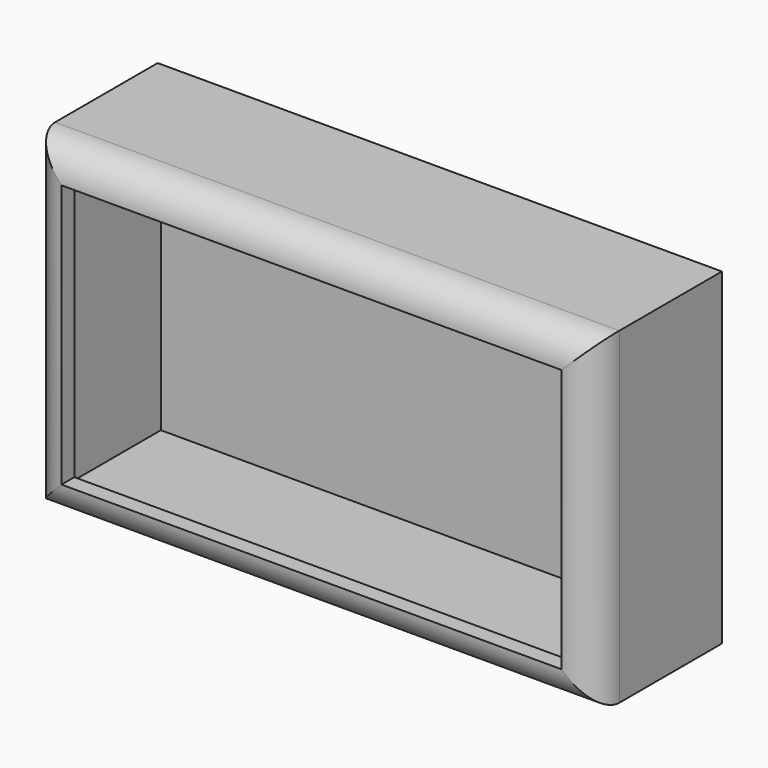
from build123d import *

# Parameters (mm, degrees)
F0_W     = 88
F0_H     = 51.0847450688
F1_DEPTH = 25
F2_R     = 5
F3_T     = -2.5


# Not quite as in the source:
# - a shell that OpenCascade refuses in one call is made with other operations: the cavity is built on its own and cut out


with BuildPart() as f1:
    # F0 (on Front) → F1 (new body)
    with BuildSketch(Plane.XZ):
        with Locations((-8.0169501303, 25.5423725344)):
            Rectangle(F0_W, F0_H)
    extrude(amount=F1_DEPTH)

    # F2
    f2_edges = [f1.edges().sort_by_distance(p)[0] for p in [
        (-52.01695, -25, 25.542373),
        (-8.01695, -25, 0),
        (35.98305, -25, 25.542373),
        (-8.01695, -25, 51.084745),
    ]]
    fillet(f2_edges, radius=F2_R)

    # F3: a shell. OpenCascade refuses it in one call, so the cavity is built on its own and cut out:
    # the body offset inwards by the wall thickness, plus a prism from it out through each open face.
    f3_core = offset(f1.part, amount=F3_T, mode=Mode.PRIVATE)
    f3_exits = [f3_core.faces().sort_by_distance(p)[0] for p in [
        (-8.01695, -22.5, 25.542373),
    ]]
    add(f3_core, mode=Mode.SUBTRACT)
    extrude(f3_exits, amount=-F3_T, mode=Mode.SUBTRACT)


solid = f1.part
